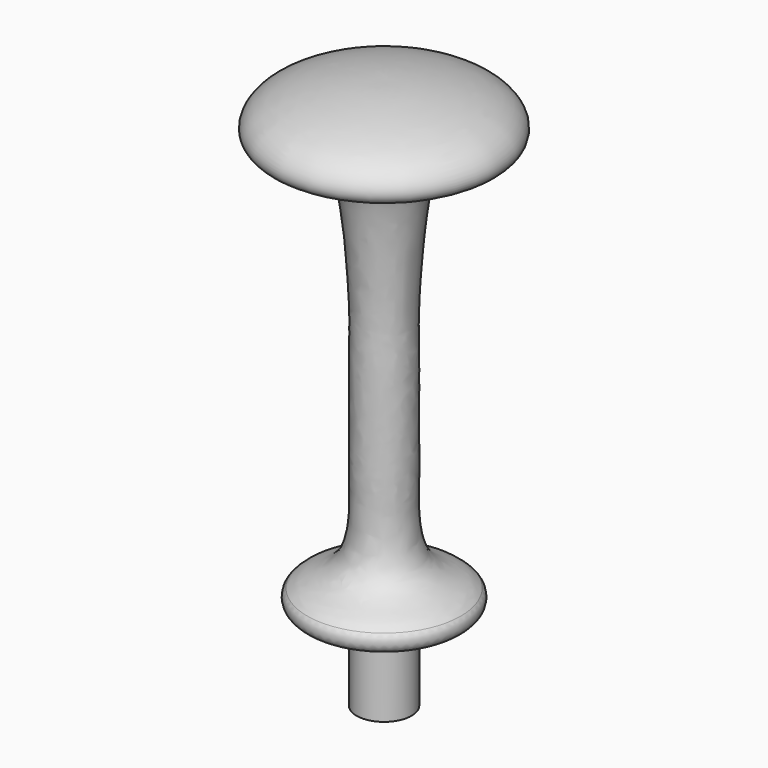
from build123d import *

# Parameters (mm, degrees)
F3_R     = 2.54
F4_R     = 1.5875
F5_DEPTH = 19.05


# Not quite as in the source:
# - a fillet or chamfer that OpenCascade refuses, or shapes differently, is made with other operations: its cross-section is extruded or revolved along the edge and cut away or added


with BuildPart() as f1:
    # F0 (on Front) → F1 (revolve)
    with BuildSketch(Plane.XZ):
        with BuildLine():
            Line((-6.35, 0), (0, 0))
            Line((0, 0), (0, 127))
            add(Edge.make_bspline(
                [(-19.05, 22.225), (-17.9092399161, 24.1243307144), (-15.1161812924, 25.9633771173), (-5.8978034426, 29.5192079863), (-6.4536835474, 46.8879752408), (-6.2975557616, 54.0864604526), (-6.4421027783, 73.7577790473), (-6.0833839935, 80.8464435843), (-7.7793010408, 104.9393920253), (-11.0195601855, 113.7080288514), (-27.7898843554, 113.3853824931), (-25.0886500303, 123.7114705068), (-6.2186074955, 127.1604456256), (-1.7664065095, 126.9919508964), (0, 127)],
                knots=[0, 0, 0, 0, 0.0586147571, 0.131001305, 0.2292294673, 0.3032893264, 0.4098539345, 0.483783041, 0.6045832141, 0.6781801825, 0.768311088, 0.8290674945, 0.9368345939, 1, 1, 1, 1], degree=3))
            Line((-19.05, 22.225), (-19.05, 19.05))
            Line((-19.05, 19.05), (-6.35, 19.05))
            Line((-6.35, 19.05), (-6.35, 0))
        make_face()
    revolve(axis=Axis((0, 0, 63.5), (0, 0, 1)))

    # F2: fillet of radius 5.08 on 1 edges, made by hand

    # F2_s1 → F2_t2 (revolve, cut)
    with BuildSketch(Plane.XZ):
        with BuildLine():
            ThreePointArc((-19.05, 22.225), (-17.1805202921, 19.9178865162), (-14.3407139607, 19.05))
            Line((-14.3407139607, 19.05), (-19.05, 19.05))
            Line((-19.05, 19.05), (-19.05, 22.225))
        make_face()
    revolve(axis=Axis((0, 0, 19.05), (0, 0, 1)), mode=Mode.SUBTRACT)

    # F3
    f3_edges = [f1.edges().sort_by_distance(p)[0] for p in [
        (19.05, 0, 22.225),
    ]]
    fillet(f3_edges, radius=F3_R)

    # F4 (on face) → F5 (cut)
    with BuildSketch(Plane(origin=(0, 0, 0), x_dir=(1, 0, 0), z_dir=(0, 0, -1))):
        Circle(F4_R)
    extrude(amount=-F5_DEPTH, mode=Mode.SUBTRACT)


solid = f1.part
